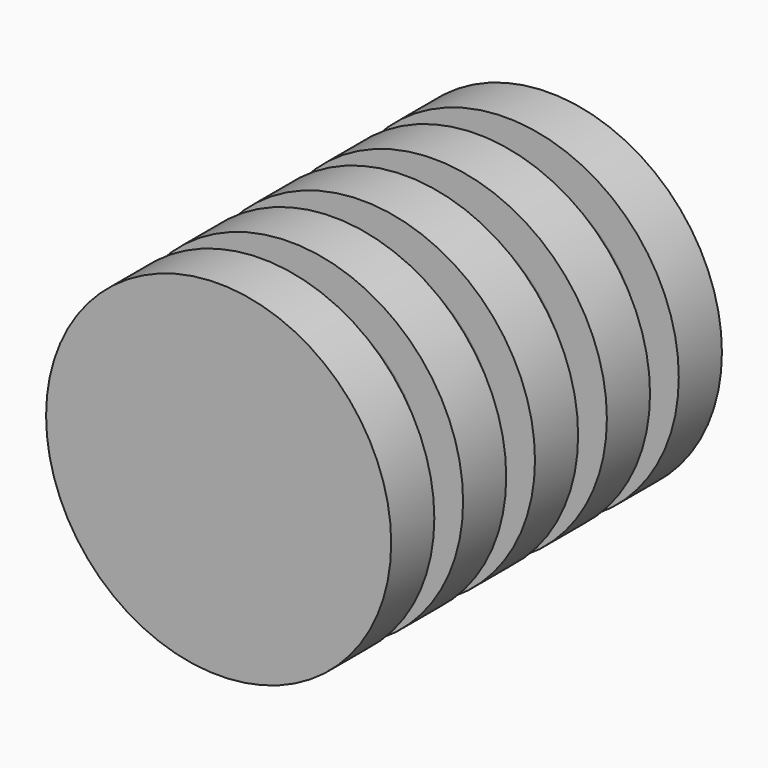
from build123d import *

# Parameters (mm, degrees)
F2_R = 0.99999


# Not quite as in the source:
# - a fillet or chamfer is up to 0.001 mm smaller than in the source, because OpenCascade refuses the exact size
# - a feature names something its author has since deleted; it is built from what else it names


with BuildPart() as f1:
    # F0 (on Top) → F1 (revolve)
    with BuildSketch(Plane.XY):
        Polygon((0, 23), (0, 0), (9.6, 0), (9.6, 3), (6.6, 3), (6.6, 5), (9.6, 5), (9.6, 8), (6.6, 8), (6.6, 10), (9.6, 10), (9.6, 13), (6.6, 13), (6.6, 15), (9.6, 15), (9.6, 18), (6.6, 18), (6.6, 20), (9.6, 20), (9.6, 23), align=None)
    revolve(axis=Axis((0, 11.5, 0), (0, 1, 0)))

    # F2 (radius 1 in the source; OpenCascade refuses exactly that, so slightly less here)
    f2_edges = [f1.edges().sort_by_distance(p)[0] for p in [
        (-6.6, 20, 0),
        (-6.6, 15, 0),
        (-6.6, 10, 0),
        (-6.6, 5, 0),
        (-6.6, 3, 0),
        (-6.6, 8, 0),
        (-6.6, 13, 0),
        (-6.6, 18, 0),
    ]]
    fillet(f2_edges, radius=F2_R)


solid = f1.part
